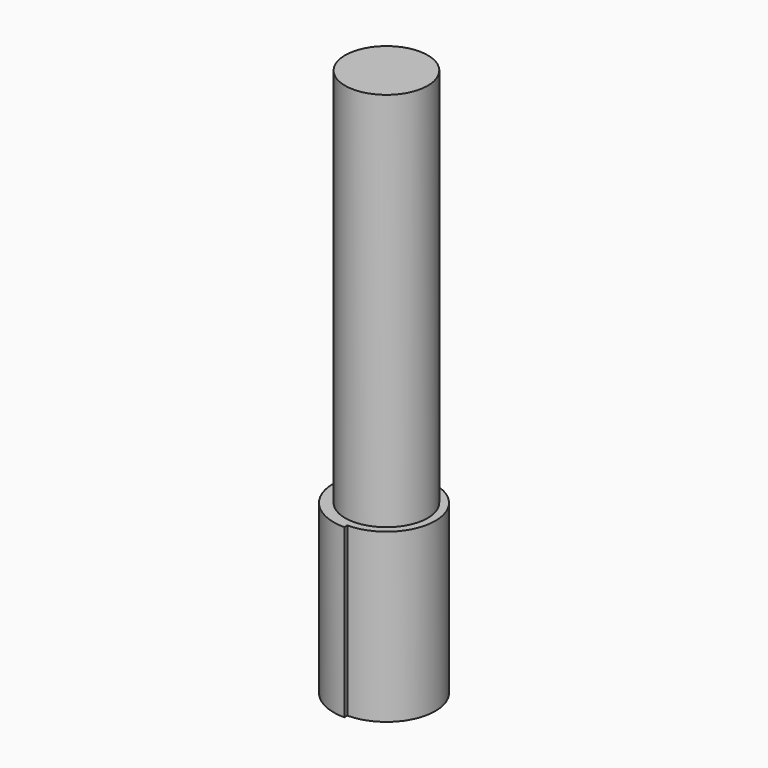
from build123d import *
from build123d import SkipClean  # not in build123d's __all__

# Parameters (mm, degrees)
F1_ANGLE_BACK = 90
F1_ANGLE      = 180
F3_ANGLE_BACK = 90
F3_ANGLE      = 180


with BuildPart() as f1:
    # F0 (on Front) → F1 (revolve)
    with BuildSketch(Plane.XZ, mode=Mode.PRIVATE) as f1_sk:
        Polygon((5.425, 0), (0, 0), (0, -72), (6.425, -72), (6.425, -50), (5.425, -50), align=None)
    revolve(f1_sk.sketch.rotate(Axis((0, 0, -36), (0, 0, 1)), -F1_ANGLE_BACK), axis=Axis((0, 0, -36), (0, 0, 1)), revolution_arc=F1_ANGLE)

    # F2 (on Front) → F3 (revolve)
    with BuildSketch(Plane.XZ, mode=Mode.PRIVATE) as f3_sk:
        Polygon((0, -72), (0, 0), (-5.425, 0), (-5.425, -50), (-6.925, -50), (-6.925, -72), align=None)
    revolve(f3_sk.sketch.rotate(Axis((0, 0, -36), (0, 0, 1)), -F3_ANGLE_BACK), axis=Axis((0, 0, -36), (0, 0, 1)), revolution_arc=F3_ANGLE)


solid = f1.part
